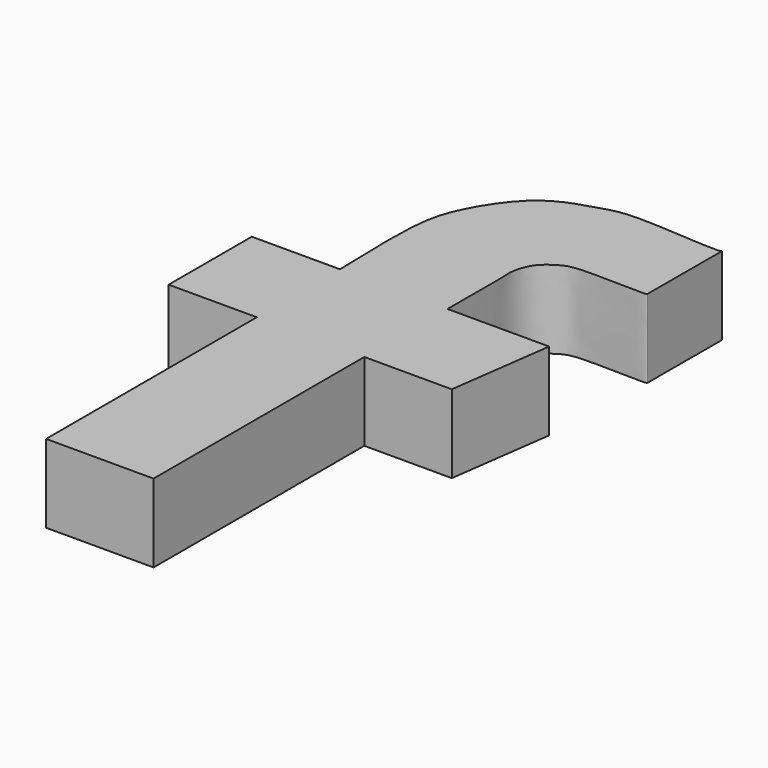
from build123d import *

# Parameters (mm, degrees)
F1_DEPTH = 10


# Not quite as in the source:
# - a feature of the source that left no trace in its solid (it failed there, or was rolled back) is left out


with BuildPart() as f1:
    # F0 (on Top) → F1 (new body)
    with BuildSketch(Plane.XY):
        with BuildLine():
            Line((3.9948658086, -37.9601344466), (3.9948658086, -4.2929993942))
            Line((3.9948658086, -4.2929993942), (15.1785674321, -4.2929993942))
            Line((15.1785674321, -4.2929993942), (16.9891585852, 8.9931276855))
            Line((16.9891585852, 8.9931276855), (3.9948658086, 8.9907931754))
            add(Edge.make_bspline(
                [(3.9948658086, 8.9907931754), (4.027739325, 12.1601402389), (4.0778996896, 16.9961183151), (3.8334442726, 19.3064516597), (4.635462537, 21.9035751502), (6.7271846954, 23.3618004084), (8.5168941226, 24.2723359095), (17.4967051794, 23.6923218521), (17.5463882122, 23.9686446329), (17.5514686853, 23.9969007671)],
                knots=[0, 0, 0, 0, 0.232803278, 0.3552250751, 0.4838975823, 0.6064647181, 0.7356243424, 0.9729655512, 1, 1, 1, 1], degree=3))
            Line((17.5514686853, 23.9969007671), (17.5810336279, 35.8575776823))
            add(Edge.make_bspline(
                [(-9.7417384386, 8.9907931754), (-9.8846499396, 13.6340507262), (-10.1166925595, 21.1732175473), (-8.8549206442, 25.9531324701), (-6.028707478, 30.7994848228), (-2.5777889056, 34.0867208483), (2.5751128853, 35.6122541827), (6.0884512365, 36.6764900581), (17.2638557744, 35.458509778), (17.5759933146, 35.8452261681), (17.5810336279, 35.8575776823)],
                knots=[0, 0, 0, 0, 0.1927092977, 0.3128983322, 0.4395299884, 0.5595460824, 0.6799631693, 0.8000187556, 0.9783779377, 0.9838927772, 0.9838927772, 0.9838927772, 0.9838927772], degree=3))
            Line((-9.7417384386, 8.9907931754), (-21.010985598, 8.9907931754))
            Line((-21.010985598, 8.9907931754), (-21.010985598, -4.2929993942))
            Line((-21.010985598, -4.2929993942), (-9.7417384386, -4.2929993942))
            Line((-9.7417384386, -4.2929993942), (-9.7417384386, -37.9601344466))
            Line((-9.7417384386, -37.9601344466), (3.9948658086, -37.9601344466))
        make_face()
    extrude(amount=F1_DEPTH)


solid = f1.part
